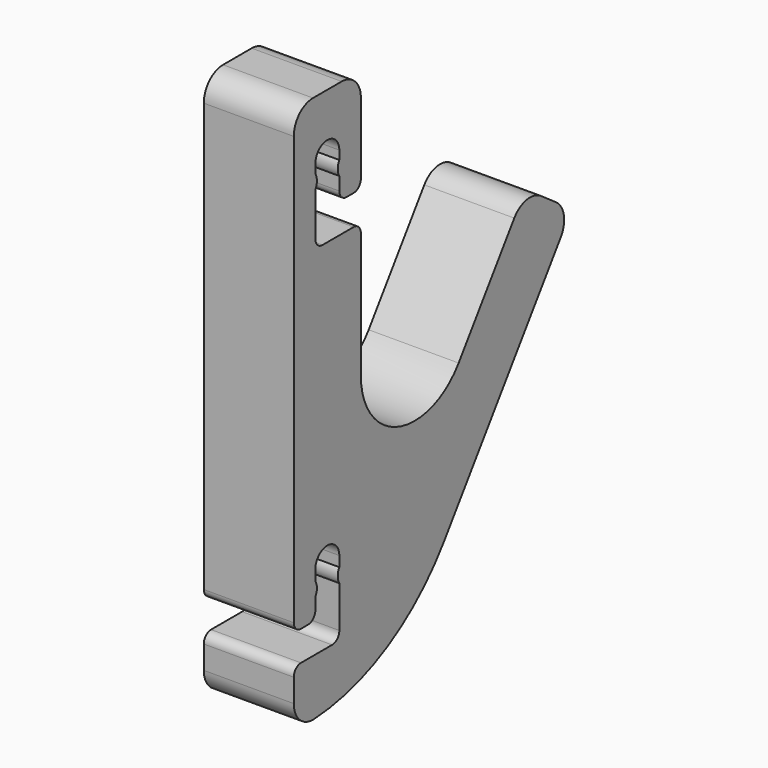
from build123d import *

# Parameters (mm, degrees)
F1_DEPTH = 3.81
F2_R     = 2.032
F4_DEPTH = 7.621
F5_R     = 0.762
F7_DEPTH = 7.62


# Not quite as in the source:
# - a feature names something its author has since deleted; it is built from what else it names


with BuildPart() as f1:
    # F0 (on Right) → F1 (new body, symmetric)
    with BuildSketch(Plane.YZ):
        with BuildLine():
            Line((0, 42.3580370843), (0, 0))
            Line((0, 0), (0, -3.979871033))
            ThreePointArc((0, -3.979871033), (8.9499402185, -2.2460183558), (15.9004898533, 3.6529251764))
            Line((15.9004898533, 3.6529251764), (29.4239599312, 22.9664420122))
            Line((29.4239599312, 22.9664420122), (24.5073227445, 26.4091084329))
            Line((24.5073227445, 26.4091084329), (17.4524241549, 16.3336690744))
            ThreePointArc((17.4524241549, 16.3336690744), (11.0805919315, 14.1707234894), (7.1017071605, 19.5972376068))
            Line((7.1017071605, 19.5972376068), (7.1017071605, 42.3580370843))
            Line((7.1017071605, 42.3580370843), (0, 42.3580370843))
        make_face()
    extrude(amount=F1_DEPTH, both=True)

    # F2
    f2_edges = [f1.edges().sort_by_distance(p)[0] for p in [
        (0, 7.101707, 42.358037),
        (0, 0, 42.358037),
        (0, 29.42396, 22.966442),
        (0, 24.507323, 26.409108),
        (0, 0, -3.979871),
    ]]
    fillet(f2_edges, radius=F2_R)

    # F3 (on face) → F4 (cut, through all)
    with BuildSketch(Plane.YZ.offset(3.81)):
        with BuildLine():
            Line((4.8208535802, 33.5311107337), (4.8208535802, 37.3411107337))
            ThreePointArc((4.8208535802, 37.3411107337), (3.5508535802, 38.6111107337), (2.2808535802, 37.3411107337))
            Line((2.2808535802, 37.3411107337), (2.2808535802, 30.9911107337))
            Line((2.2808535802, 30.9911107337), (7.1017071605, 30.9911107337))
            Line((7.1017071605, 30.9911107337), (7.1017071605, 33.5311107337))
            Line((7.1017071605, 33.5311107337), (4.8208535802, 33.5311107337))
        make_face()
        with BuildLine():
            Line((4.8208535802, 0.7651107337), (4.8208535802, 7.1151107337))
            ThreePointArc((4.8208535802, 7.1151107337), (3.5508535802, 8.3851107337), (2.2808535802, 7.1151107337))
            Line((2.2808535802, 7.1151107337), (2.2808535802, 3.3051107337))
            Line((2.2808535802, 3.3051107337), (0, 3.3051107337))
            Line((0, 3.3051107337), (0, 0.7651107337))
            Line((0, 0.7651107337), (4.8208535802, 0.7651107337))
        make_face()
    extrude(amount=-F4_DEPTH, mode=Mode.SUBTRACT)

    # F5
    f5_edges = [f1.edges().sort_by_distance(p)[0] for p in [
        (0, 4.820854, 33.531111),
        (0, 7.101707, 33.531111),
        (0, 2.280854, 30.991111),
        (0, 7.101707, 30.991111),
        (0, 0, 3.305111),
        (0, 4.820854, 0.765111),
        (0, 0, 0.765111),
        (0, 2.280854, 3.305111),
    ]]
    fillet(f5_edges, radius=F5_R)

    # F6 (on face) → F7 (join, through all)
    with BuildSketch(Plane.YZ.offset(3.81)):
        with BuildLine():
            Line((4.8208535802, 35.4121252894), (4.8208535802, 36.6062968969))
            ThreePointArc((4.8208535802, 36.6062968969), (4.6525009744, 36.0092110932), (4.8208535802, 35.4121252894))
        make_face()
        with BuildLine():
            Line((2.2808535802, 36.6062968969), (2.2808535802, 35.4121252894))
            ThreePointArc((2.2808535802, 35.4121252894), (2.4492061861, 36.0092110932), (2.2808535802, 36.6062968969))
        make_face()
        with BuildLine():
            Line((2.2808535802, 6.2474817969), (2.2808535802, 5.0533101894))
            ThreePointArc((2.2808535802, 5.0533101894), (2.4492061861, 5.6503959931), (2.2808535802, 6.2474817969))
        make_face()
        with BuildLine():
            ThreePointArc((4.8208535802, 6.2474817969), (4.6525009744, 5.6503959931), (4.8208535802, 5.0533101894))
            Line((4.8208535802, 5.0533101894), (4.8208535802, 6.2474817969))
        make_face()
    extrude(amount=-F7_DEPTH)


solid = f1.part
